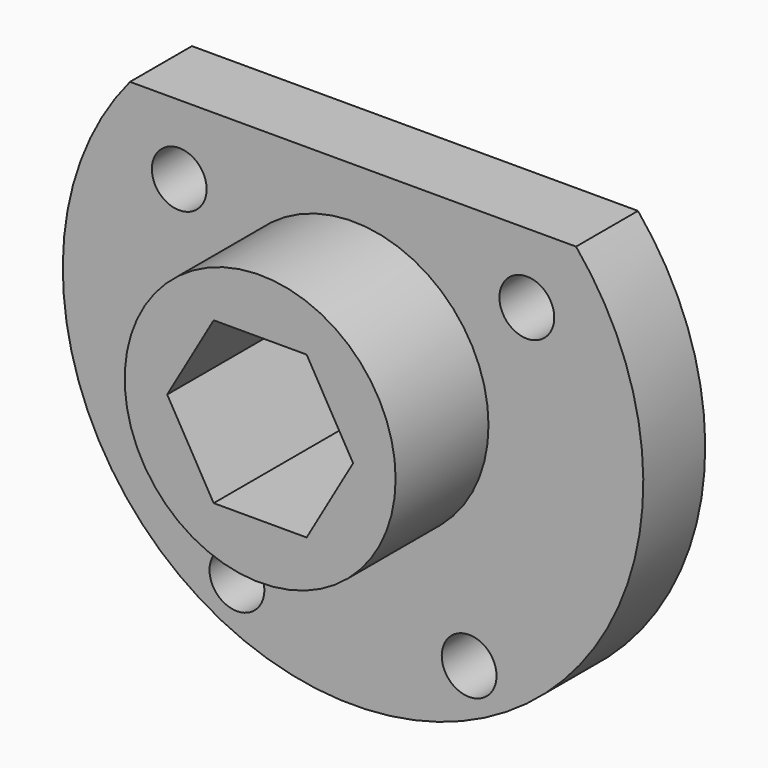
from build123d import *

# Parameters (mm, degrees)
F1_DEPTH = 6.35
F3_D     = 4.4958
F4_R     = 11.1125
F5_DEPTH = 9.525
F7_DEPTH = 15.876


with BuildPart() as f1:
    # F0 (on Front) → F1 (new body)
    with BuildSketch(Plane.XZ):
        with BuildLine():
            Line((18.2969275085, 15.24), (-18.2969275085, 15.24))
            ThreePointArc((-18.2969275085, 15.24), (0, -23.8125), (18.2969275085, 15.24))
        make_face()
    extrude(amount=F1_DEPTH)

    # F3 (through all)
    with Locations(Plane.XZ.offset(6.35)):
        with Locations((-14.2575098316, 9.525), (14.2575098316, 9.525), (9.525, -17.8901402442), (-9.525, -17.8901402442)):
            Hole(F3_D / 2)

    # F4 (on face) → F5 (join)
    with BuildSketch(Plane.XZ.offset(6.35)):
        Circle(F4_R)
    extrude(amount=F5_DEPTH)

    # F6 (on face) → F7 (cut, through all)
    with BuildSketch(Plane.XZ.offset(15.875)):
        Polygon((3.8128211777, -6.604), (7.6256423555, 0), (3.8128211777, 6.604), (-3.8128211777, 6.604), (-7.6256423555, 0), (-3.8128211777, -6.604), align=None)
    extrude(amount=-F7_DEPTH, mode=Mode.SUBTRACT)


solid = f1.part
